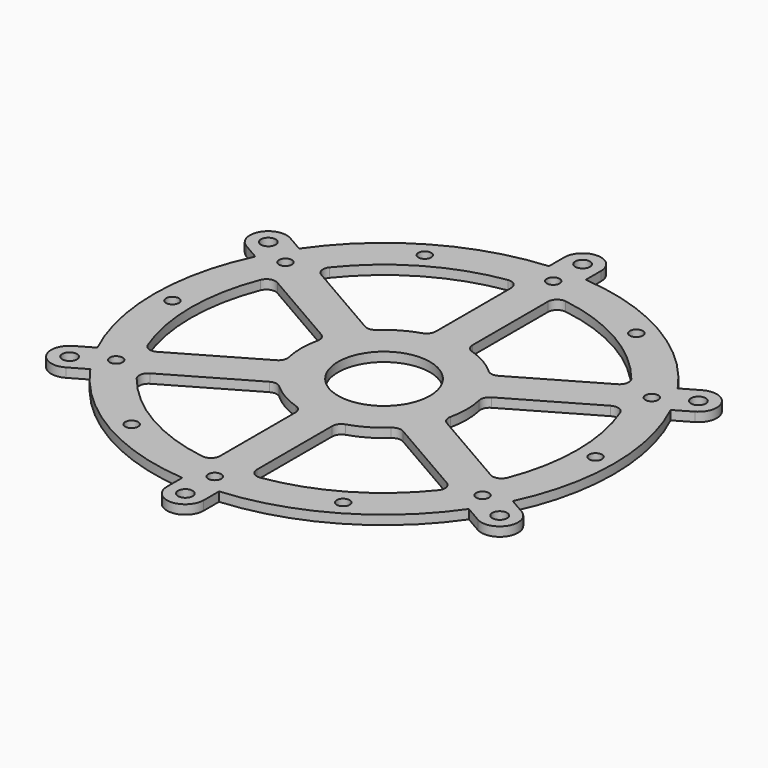
from build123d import *

# Parameters (mm, degrees)
F1_R             = 125
F4_DEPTH         = 5
F5_DEPTH         = 5
F5_COPIES_COUNT  = 6
F6_DEPTH         = 5
F6_COPIES_COUNT  = 6
F0_R             = 25
F7_DEPTH         = 25
F8_R             = 4
F9_DEPTH         = 5
F9_COPIES_COUNT  = 6
F10_R            = 3.5
F11_DEPTH        = 5
F11_COPIES_COUNT = 12


# Not quite as in the source:
# - a pattern or mirror of a feature is missing from the dataset's text; its kind, count and spacing are read off the source's solid


with BuildPart() as f4:
    # F1 (on Top) → F4 (new body)
    with BuildSketch(Plane.XY):
        Circle(F1_R)
    extrude(amount=-F4_DEPTH)

    # F2 (on Top) → F5 (cut, through all)
    with BuildSketch(Plane.XY):
        with BuildLine():
            ThreePointArc((15.75, 103.8120296497), (11.7403987974, 102.6600373885), (10, 98.8685996664))
            Line((10, 98.8685996664), (10, 47.6969600708))
            ThreePointArc((10, 47.6969600708), (10.9688711259, 44.7389201793), (13.5, 42.9272640638))
            ThreePointArc((13.5, 42.9272640638), (22.5, 38.9711431703), (30.4261011942, 33.154974983))
            ThreePointArc((30.4261011942, 33.154974983), (33.2606058502, 31.8687811355), (36.3067791046, 32.5087340733))
            Line((36.3067791046, 32.5087340733), (80.6227189477, 58.0945538711))
            ThreePointArc((80.6227189477, 58.0945538711), (83.0360009332, 61.4975023033), (82.0288548951, 65.5459149345))
            ThreePointArc((82.0288548951, 65.5459149345), (52.5, 90.9326673974), (15.75, 103.8120296497))
        make_face()
    f5 = extrude(amount=-F5_DEPTH, mode=Mode.SUBTRACT)

    # F5_copies: F5 ×6 about axis
    f5_copies_axis = Axis((0, 0, 0), (0, 0, 1))
    for i in range(1, F5_COPIES_COUNT):
        add(f5.rotate(f5_copies_axis, i * 360 / F5_COPIES_COUNT), mode=Mode.SUBTRACT)

    # F3 (on Top) → F6 (join, through all)
    with BuildSketch(Plane.XY):
        with BuildLine():
            Line((-10, 135), (-10, 120))
            Line((-10, 120), (10, 120))
            Line((10, 120), (10, 135))
            ThreePointArc((10, 135), (0, 145), (-10, 135))
        make_face()
    f6 = extrude(amount=-F6_DEPTH)

    # F6_copies: F6 ×6 about axis
    f6_copies_axis = Axis((0, 0, 0), (0, 0, 1))
    for i in range(1, F6_COPIES_COUNT):
        add(f6.rotate(f6_copies_axis, i * 360 / F6_COPIES_COUNT))

    # F0 (on Top) → F7 (cut)
    with BuildSketch(Plane.XY):
        Circle(F0_R)
    extrude(amount=-F7_DEPTH, mode=Mode.SUBTRACT)

    # F8 (on Top) → F9 (cut, through all)
    with BuildSketch(Plane.XY):
        with Locations((0, 135)):
            Circle(F8_R)
    f9 = extrude(amount=-F9_DEPTH, mode=Mode.SUBTRACT)

    # F9_copies: F9 ×6 about axis
    f9_copies_axis = Axis((0, 0, 0), (0, 0, 1))
    for i in range(1, F9_COPIES_COUNT):
        add(f9.rotate(f9_copies_axis, i * 360 / F9_COPIES_COUNT), mode=Mode.SUBTRACT)

    # F10 (on Top) → F11 (cut, through all)
    with BuildSketch(Plane.XY):
        with Locations((0, 115)):
            Circle(F10_R)
    f11 = extrude(amount=-F11_DEPTH, mode=Mode.SUBTRACT)

    # F11_copies: F11 ×12 about axis
    f11_copies_axis = Axis((0, 0, 0), (0, 0, 1))
    for i in range(1, F11_COPIES_COUNT):
        add(f11.rotate(f11_copies_axis, i * 360 / F11_COPIES_COUNT), mode=Mode.SUBTRACT)


solid = f4.part
